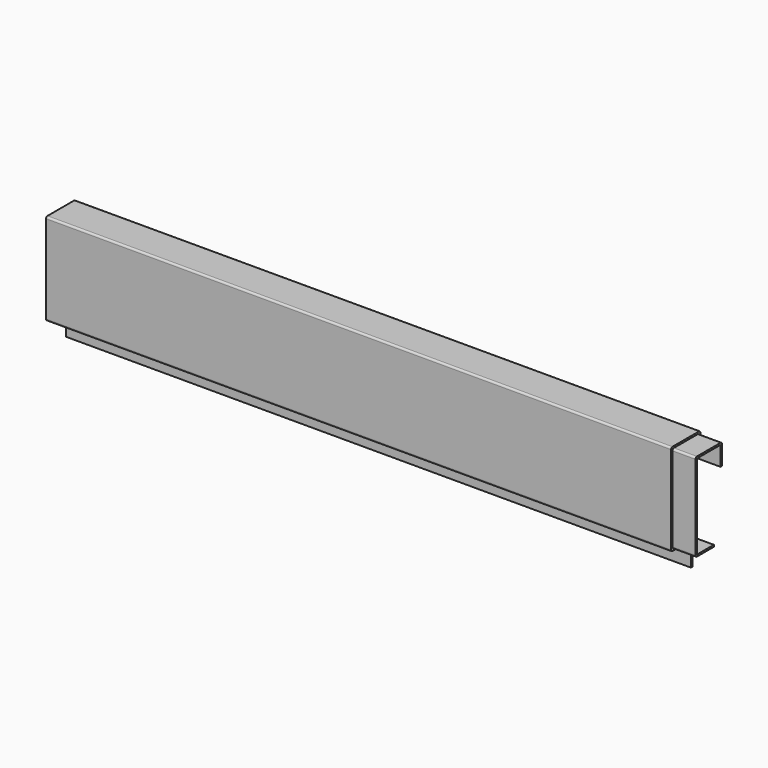
from build123d import *

# Parameters (mm, degrees)
F1_DEPTH      = 680
F3_D          = 5
F4_R          = 2
F6_DEPTH      = 25
F6_DEPTH_BACK = 25


# Not quite as in the source:
# - a feature names something its author has since deleted; it is built from what else it names


with BuildPart() as f1:
    # F0 (on Right) → F1 (new body)
    with BuildSketch(Plane.YZ):
        Polygon((-18.8378913403, 177.8021101952), (-18.8378913403, 154.8021101952), (-16.8378913403, 154.8021101952), (-16.8378913403, 179.8021101952), (-56.8378913403, 179.8021101952), (-56.8378913403, 79.8021101952), (-29.8378913403, 79.8021101952), (-29.8378913403, 53.8021101952), (-27.8378913403, 53.8021101952), (-27.8378913403, 81.8021101952), (-54.8378913403, 81.8021101952), (-54.8378913403, 177.8021101952), align=None)
    extrude(amount=F1_DEPTH)

    # F3 (through all)
    with Locations(Plane.XZ.offset(29.8378913403)):
        with Locations((580, 66.8021101952), (100, 66.8021101952)):
            Hole(F3_D / 2)

    # F4
    f4_edges = [f1.edges().sort_by_distance(p)[0] for p in [
        (340, -56.837891, 179.80211),
        (340, -16.837891, 179.80211),
        (340, -56.837891, 79.80211),
        (340, -27.837891, 81.80211),
        (340, -54.837891, 81.80211),
        (340, -29.837891, 79.80211),
        (340, -18.837891, 177.80211),
        (340, -54.837891, 177.80211),
    ]]
    fillet(f4_edges, radius=F4_R)

    # F5 (on face) → F6 (join, two sides)
    with BuildSketch(Plane.YZ.offset(680)) as f6_sk:
        with BuildLine():
            Line((-20.8378913403, 154.8021101952), (-18.8378913403, 154.8021101952))
            Line((-18.8378913403, 154.8021101952), (-18.8378913403, 175.8021101952))
            ThreePointArc((-18.8378913403, 175.8021101952), (-19.4236777779, 177.2163237575), (-20.8378913403, 177.8021101952))
            Line((-20.8378913403, 177.8021101952), (-52.8378913403, 177.8021101952))
            ThreePointArc((-52.8378913403, 177.8021101952), (-54.2521049026, 177.2163237575), (-54.8378913403, 175.8021101952))
            Line((-54.8378913403, 175.8021101952), (-54.8378913403, 83.8021101952))
            ThreePointArc((-54.8378913403, 83.8021101952), (-54.2521049026, 82.3878966328), (-52.8378913403, 81.8021101952))
            Line((-52.8378913403, 81.8021101952), (-29.8378913403, 81.8021101952))
            Line((-29.8378913403, 81.8021101952), (-29.8378913403, 83.8021101952))
            Line((-29.8378913403, 83.8021101952), (-52.8378913403, 83.8021101952))
            Line((-52.8378913403, 83.8021101952), (-52.8378913403, 175.8021101952))
            Line((-52.8378913403, 175.8021101952), (-20.8378913403, 175.8021101952))
            Line((-20.8378913403, 175.8021101952), (-20.8378913403, 154.8021101952))
        make_face()
    extrude(amount=F6_DEPTH)
    extrude(f6_sk.sketch, amount=-F6_DEPTH_BACK)


solid = f1.part
